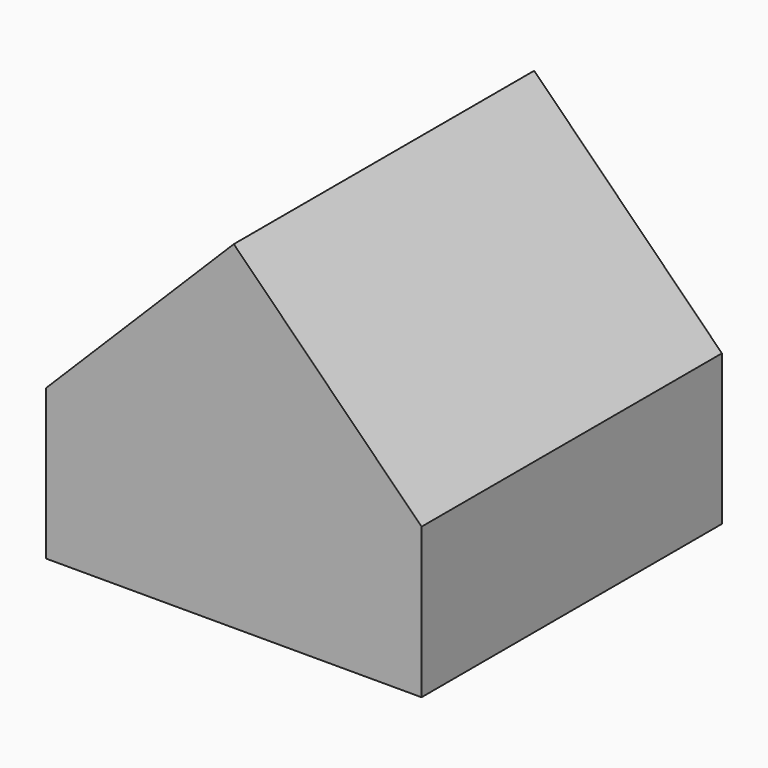
from build123d import *

# Parameters (mm, degrees)
F0_W     = 50
F0_H     = 50
F0_W_2   = 40
F0_H_2   = 40
F1_DEPTH = 20
F2_W     = 50
F2_H     = 50
F3_DEPTH = 25
F4_SIZE  = 24.99999


# Not quite as in the source:
# - a fillet or chamfer is up to 0.001 mm smaller than in the source, because OpenCascade refuses the exact size


with BuildPart() as f1:
    # F0 (on Top) → F1 (new body)
    with BuildSketch(Plane.XY):
        with Locations((25, 25)):
            Rectangle(F0_W, F0_H)
        with Locations((25, 25)):
            Rectangle(F0_W_2, F0_H_2, mode=Mode.SUBTRACT)
    extrude(amount=F1_DEPTH)

    # F2 (on face) → F3 (join)
    with BuildSketch(Plane.XY.offset(20)):
        with Locations((25, 25)):
            Rectangle(F2_W, F2_H)
    extrude(amount=F3_DEPTH)

    # F4 (size 25 in the source; OpenCascade refuses exactly that, so slightly less here)
    f4_edges = [f1.edges().sort_by_distance(p)[0] for p in [
        (0, 25, 45),
        (50, 25, 45),
    ]]
    chamfer(f4_edges, length=F4_SIZE)


solid = f1.part
